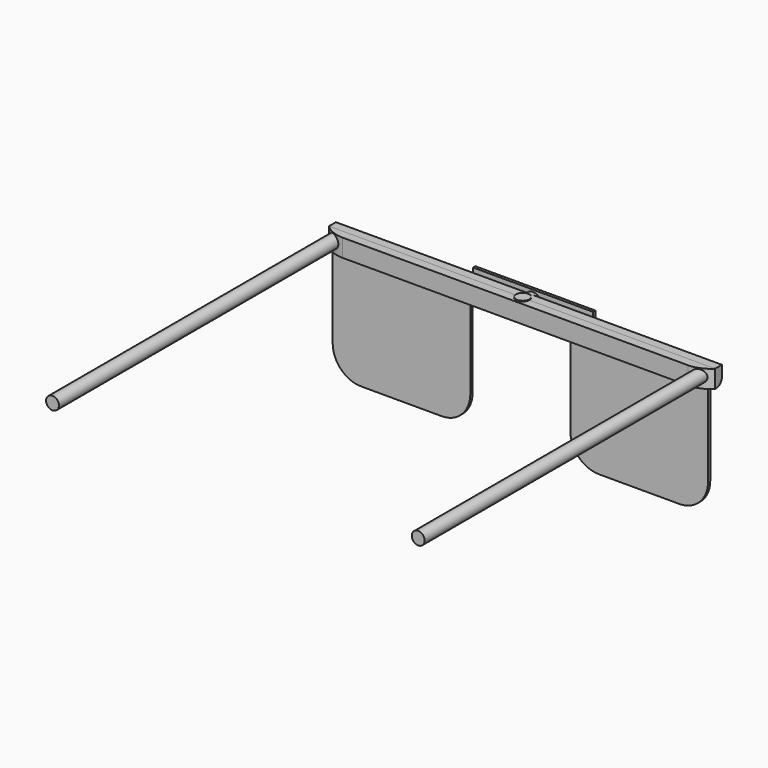
from build123d import *

# Parameters (mm, degrees)
F0_W        = 24.4474970783
F0_H        = 21.6693738201
F1_DEPTH    = 0.508
F2_W        = 68.58
F2_H        = 3.1658634543
F3_DEPTH    = 1.524
F4_DEPTH    = 1.524
F5_R        = 5.08
F5_2_R      = 5.08
F6_R        = 1.143
F7_DEPTH    = 63.5
F8_R        = 1.27
F9_T1_DEPTH = 21.3050916628
F10_R       = 1.5092579777
F11_DEPTH   = 2.286
F12_W       = 21.3444312233
F12_H       = 3.81
F12_R       = 1.5092579777
F13_DEPTH   = 0.508
F15_DEPTH   = 0.127


# Not quite as in the source:
# - a fillet or chamfer that OpenCascade refuses, or shapes differently, is made with other operations: its cross-section is extruded or revolved along the edge and cut away or added


with BuildPart() as f1:
    # F0 (on Front) → F1 (new body)
    with BuildSketch(Plane.XZ):
        with Locations((-21.1137485391, 10.83468691)):
            Rectangle(F0_W, F0_H)
    extrude(amount=F1_DEPTH)

    # F5
    f5_edges = [f1.edges().sort_by_distance(p)[0] for p in [
        (-8.89, -0.254, 0),
        (-33.337497, -0.254, 0),
    ]]
    fillet(f5_edges, radius=F5_R)


with BuildPart() as f1b:
    # F0 (on Front) → F1, piece 2 (new body)
    with BuildSketch(Plane.XZ):
        with Locations((21.1137485391, 10.83468691)):
            Rectangle(F0_W, F0_H)
    extrude(amount=F1_DEPTH)

    # F5#2
    f5_2_edges = [f1b.edges().sort_by_distance(p)[0] for p in [
        (8.89, -0.254, 0),
        (33.337497, -0.254, 0),
    ]]
    fillet(f5_2_edges, radius=F5_2_R)


with BuildPart() as f3:
    # F2 (on Front) → F3 (new body)
    with BuildSketch(Plane.XZ):
        with Locations((-0.1027890062, 21.2976261973)):
            Rectangle(F2_W, F2_H)
    extrude(amount=F3_DEPTH)


with BuildPart() as f4:
    # F4 (new): a face of the model
    f4_faces = [f3.part.faces().sort_by_distance(p)[0] for p in [
        (-0.1027890062, 0, 21.2976261973),
    ]]
    extrude(f4_faces, amount=F4_DEPTH)

    # F8
    f8_edges = [f4.edges().sort_by_distance(p)[0] for p in [
        (-0.102789, 1.524, 19.714694),
    ]]
    fillet(f8_edges, radius=F8_R)


with BuildPart() as f7:
    # F6 (on Front) → F7 (new body)
    with BuildSketch(Plane.XZ):
        with Locations((32.2467535734, 21.5597579245)):
            Circle(F6_R)
    extrude(amount=F7_DEPTH)


with BuildPart() as f7b:
    # F6 (on Front) → F7, piece 2 (new body)
    with BuildSketch(Plane.XZ):
        with Locations((-32.7254012227, 21.5597579245)):
            Circle(F6_R)
    extrude(amount=F7_DEPTH)


with BuildPart() as f3_1:
    add(f3.part)

    # F9: fillet of radius 5.08 on 2 edges, made by hand

    # F9_s2 → F9_t1 (cut)
    with BuildSketch(Plane.XY.offset(10.6450803659)):
        with BuildLine():
            ThreePointArc((34.1872109938, 0), (32.5268408919, -1.1275285843), (30.5593653521, -1.524))
            Line((30.5593653521, -1.524), (34.1872109938, -1.524))
            Line((34.1872109938, -1.524), (34.1872109938, 0))
        make_face()
        with BuildLine():
            ThreePointArc((-34.3927890062, 0), (-32.7324189044, -1.1275285843), (-30.7649433645, -1.524))
            Line((-30.7649433645, -1.524), (-34.3927890062, -1.524))
            Line((-34.3927890062, -1.524), (-34.3927890062, 0))
        make_face()
    extrude(amount=F9_T1_DEPTH, mode=Mode.SUBTRACT)


with BuildPart() as f11:
    # F10 (on Front) → F11 (new body)
    with BuildSketch(Plane.XZ):
        with Locations((0, 21.3380698115)):
            Circle(F10_R)
    extrude(amount=-F11_DEPTH)


with BuildPart() as f13:
    # F12 (on face) → F13 (new body)
    with BuildSketch(Plane(origin=(0, 2.286, 0), x_dir=(-1, 0, 0), z_dir=(0, 1, 0))):
        with Locations((-0.0235047191, 21.2976261973)):
            Rectangle(F12_W, F12_H)
        with Locations((0, 21.3380698115)):
            Circle(F12_R, mode=Mode.SUBTRACT)
        with Locations((0, 21.3380698115)):
            Circle(F12_R)
    extrude(amount=F13_DEPTH)


with BuildPart() as f15:
    # F14 (on face) → F15 (new body)
    with BuildSketch(Plane.XY.offset(22.8805579245)):
        with BuildLine():
            Line((-1.1864949831, 0), (1.1864949831, 0))
            ThreePointArc((1.1864949831, 0), (0, 1.1864949831), (-1.1864949831, 0))
        make_face()
        with BuildLine():
            ThreePointArc((-1.1864949831, 0), (0, -1.1864949831), (1.1864949831, 0))
            Line((1.1864949831, 0), (-1.1864949831, 0))
        make_face()
    extrude(amount=F15_DEPTH)


solid = Compound([f1.part, f1b.part, f4.part, f7.part, f7b.part, f3_1.part, f11.part, f13.part, f15.part])
